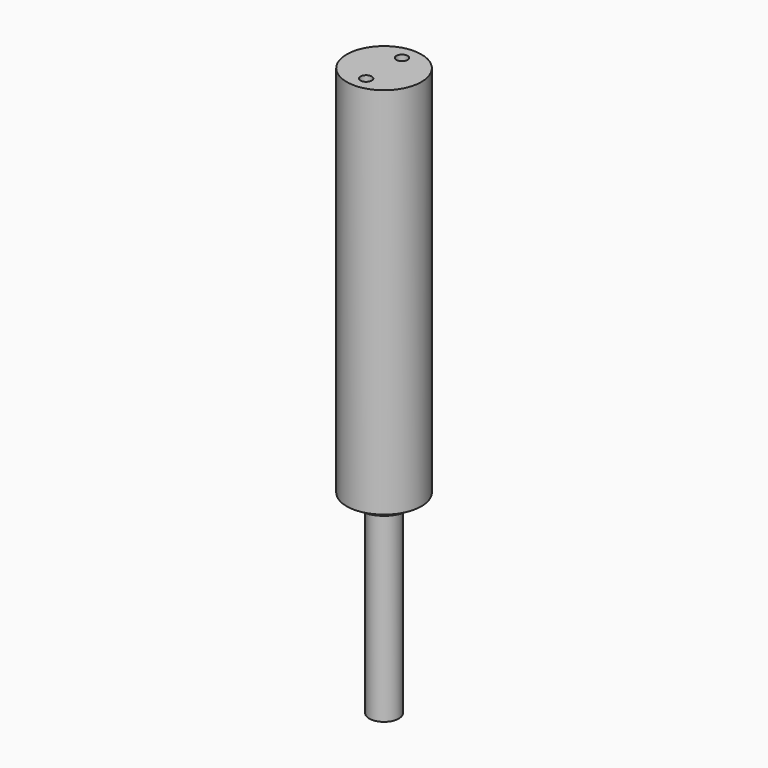
from build123d import *

# Parameters (mm, degrees)
F0_R     = 3.95
F1_DEPTH = 50
F2_R     = 6.75
F2_R_2   = 3.95
F3_DEPTH = 2
F4_R     = 10
F4_R_2   = 6.75
F5_DEPTH = 100
F6_R     = 1.5
F7_DEPTH = 10


with BuildPart() as f1:
    # F0 (on Top) → F1 (new body)
    with BuildSketch(Plane.XY):
        Circle(F0_R)
    extrude(amount=F1_DEPTH)

    # F2 (on face) → F3 (join)
    with BuildSketch(Plane.XY.offset(50)):
        Circle(F2_R)
        Circle(F2_R_2, mode=Mode.SUBTRACT)
        Circle(F2_R_2)
    extrude(amount=F3_DEPTH)

    # F4 (on face) → F5 (join)
    with BuildSketch(Plane.XY.offset(52)):
        Circle(F4_R)
        Circle(F4_R_2, mode=Mode.SUBTRACT)
        Circle(F4_R_2)
    extrude(amount=F5_DEPTH)

    # F6 (on face) → F7 (cut)
    with BuildSketch(Plane.XY.offset(152)):
        with Locations((0, 6)):
            Circle(F6_R)
        with Locations((0, -6)):
            Circle(F6_R)
    extrude(amount=-F7_DEPTH, mode=Mode.SUBTRACT)


solid = f1.part
